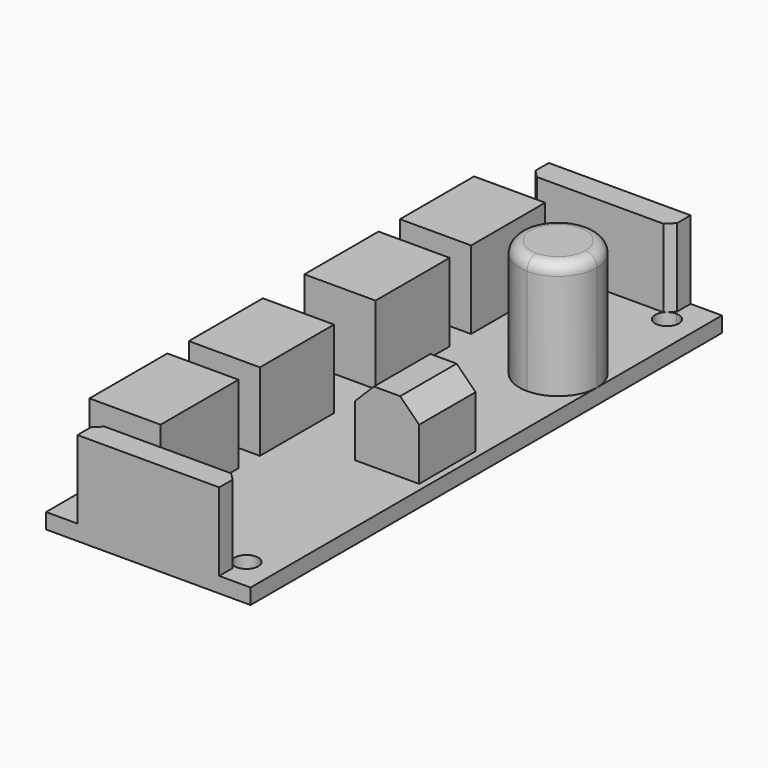
from build123d import *

# Parameters (mm, degrees)
F0_W         = 21.59
F0_H         = 62.21
F1_DEPTH     = 1.63
F4_DEPTH     = 12.34
F5_DEPTH     = 7.5
F2_R         = 1.25
F6_DEPTH     = 25
F7_SIZE      = 2
F8_R         = 1.2071067812
F10_DEPTH    = 8.23
F12_DEPTH    = 8.23
F13_T1_DEPTH = 10.2873463904
F14_W        = 7.51
F14_H        = 2.83
F14_H_2      = 5.48
F15_DEPTH    = 8.23


# Not quite as in the source:
# - a fillet or chamfer that OpenCascade refuses, or shapes differently, is made with other operations: its cross-section is extruded or revolved along the edge and cut away or added


with BuildPart() as f1:
    # F0 (on Top) → F1 (new body)
    with BuildSketch(Plane.XY):
        Rectangle(F0_W, F0_H)
    extrude(amount=F1_DEPTH)

    # F3 (on face) → F4 (join)
    with BuildSketch(Plane.XY.offset(1.63)):
        with BuildLine():
            ThreePointArc((10.7950629295, 14.605), (9.5971296646, 17.4970667351), (6.7050629295, 18.695))
            ThreePointArc((6.7050629295, 18.695), (2.6150629295, 14.605), (6.7050629295, 10.515))
            ThreePointArc((6.7050629295, 10.515), (9.5971296646, 11.7129332649), (10.7950629295, 14.605))
        make_face()
    extrude(amount=F4_DEPTH)

    # F3 (on face) → F5 (join)
    with BuildSketch(Plane.XY.offset(1.63)):
        Polygon((10.0900629295, -0.525), (6.7050629295, -0.525), (3.3200629295, -0.525), (3.3200629295, -7.975), (10.0900629295, -7.975), align=None)
    extrude(amount=F5_DEPTH)

    # F2 (on face) → F6 (cut)
    with BuildSketch(Plane.XY.offset(1.63)):
        with BuildLine():
            ThreePointArc((7.675, 29.005), (6.7911165235, 26.8711165235), (8.925, 27.755))
            Line((8.925, 27.755), (7.675, 27.755))
            Line((7.675, 27.755), (7.675, 29.005))
        make_face()
        with BuildLine():
            Line((7.675, 27.755), (8.925, 27.755))
            ThreePointArc((8.925, 27.755), (8.5588834765, 28.6388834765), (7.675, 29.005))
            Line((7.675, 29.005), (7.675, 27.755))
        make_face()
        with Locations((-7.675, 27.755)):
            Circle(F2_R)
        with Locations((-7.675, -27.755)):
            Circle(F2_R)
        with Locations((7.675, -27.755)):
            Circle(F2_R)
    extrude(amount=-F6_DEPTH, mode=Mode.SUBTRACT)

    # F7
    f7_edges = [f1.edges().sort_by_distance(p)[0] for p in [
        (3.320063, -4.25, 9.13),
        (10.090063, -4.25, 9.13),
    ]]
    chamfer(f7_edges, length=F7_SIZE)

    # F8
    f8_edges = [f1.edges().sort_by_distance(p)[0] for p in [
        (6.705063, 18.695, 13.97),
    ]]
    fillet(f8_edges, radius=F8_R)

    # F9 (on face) → F10 (join)
    with BuildSketch(Plane.XY.offset(1.63)):
        Polygon((-10.795, 25.38), (-10.795, 0), (-10.795, -25.38), (-3.285, -25.38), (-3.285, 25.38), align=None)
    extrude(amount=F10_DEPTH)

    # F11 (on face) → F12 (join)
    with BuildSketch(Plane.XY.offset(1.63)):
        with BuildLine():
            Line((7.485, 31.105), (0, 31.105))
            Line((0, 31.105), (-7.485, 31.105))
            Line((-7.485, 31.105), (-7.485, 28.9904756169))
            ThreePointArc((-7.485, 28.9904756169), (-7.0487343616, 28.8368000509), (-6.6982195743, 28.535))
            Line((-6.6982195743, 28.535), (6.6982195743, 28.535))
            ThreePointArc((6.6982195743, 28.535), (7.0487343616, 28.8368000509), (7.485, 28.9904756169))
            Line((7.485, 28.9904756169), (7.485, 31.105))
        make_face()
        with BuildLine():
            Line((7.485, 28.535), (7.485, 28.9904756169))
            ThreePointArc((7.485, 28.9904756169), (7.0487343616, 28.8368000509), (6.6982195743, 28.535))
            Line((6.6982195743, 28.535), (7.485, 28.535))
        make_face()
        with BuildLine():
            ThreePointArc((-6.6982195743, 28.535), (-7.0487343616, 28.8368000509), (-7.485, 28.9904756169))
            Line((-7.485, 28.9904756169), (-7.485, 28.535))
            Line((-7.485, 28.535), (-6.6982195743, 28.535))
        make_face()
        with BuildLine():
            Line((0, -31.105), (7.485, -31.105))
            Line((7.485, -31.105), (7.485, -28.9904756169))
            ThreePointArc((7.485, -28.9904756169), (7.0487343616, -28.8368000509), (6.6982195743, -28.535))
            Line((6.6982195743, -28.535), (-6.6982195743, -28.535))
            ThreePointArc((-6.6982195743, -28.535), (-7.0487343616, -28.8368000509), (-7.485, -28.9904756169))
            Line((-7.485, -28.9904756169), (-7.485, -31.105))
            Line((-7.485, -31.105), (0, -31.105))
        make_face()
        with BuildLine():
            ThreePointArc((6.6982195743, -28.535), (7.0487343616, -28.8368000509), (7.485, -28.9904756169))
            Line((7.485, -28.9904756169), (7.485, -28.535))
            Line((7.485, -28.535), (6.6982195743, -28.535))
        make_face()
        with BuildLine():
            Line((-7.485, -28.535), (-7.485, -28.9904756169))
            ThreePointArc((-7.485, -28.9904756169), (-7.0487343616, -28.8368000509), (-6.6982195743, -28.535))
            Line((-6.6982195743, -28.535), (-7.485, -28.535))
        make_face()
    extrude(amount=F12_DEPTH)

    # F13: chamfer of 0.8 on 4 edges, made by hand

    # F13_s2 → F13_t1 (cut)
    with BuildSketch(Plane.XY.offset(1.63)):
        Polygon((-7.485, 29.335), (-6.685, 28.535), (-7.485, 28.535), align=None)
        Polygon((6.685, 28.535), (7.485, 29.335), (7.485, 28.535), align=None)
        Polygon((-6.685, -28.535), (-7.485, -29.335), (-7.485, -28.535), align=None)
        Polygon((7.485, -29.335), (6.685, -28.535), (7.485, -28.535), align=None)
    extrude(amount=F13_T1_DEPTH, mode=Mode.SUBTRACT)

    # F14 (on face) → F15 (cut)
    with BuildSketch(Plane.XY.offset(9.86)):
        with Locations((-7.04, 14.185)):
            Rectangle(F14_W, F14_H)
        with Locations((-7.04, 0.25)):
            Rectangle(F14_W, F14_H_2)
        with Locations((-7.04, -13.685)):
            Rectangle(F14_W, F14_H)
    extrude(amount=-F15_DEPTH, mode=Mode.SUBTRACT)


solid = f1.part
